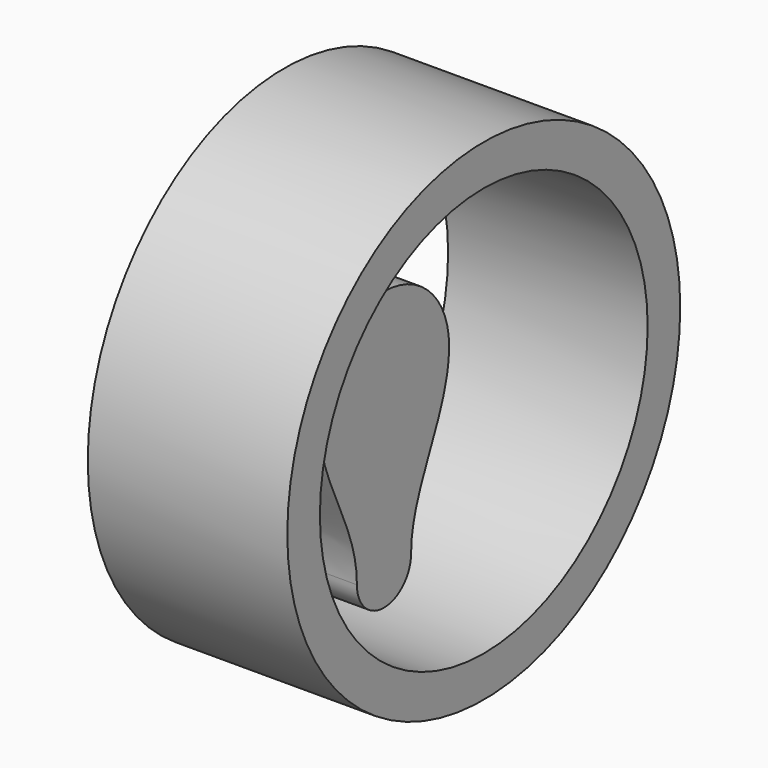
from build123d import *

# Parameters (mm, degrees)
F0_R     = 22.8209931427
F1_DEPTH = 34.544
F3_DEPTH = 51
F4_R     = 120.6073984504
F4_R_2   = 100.607397247
F5_DEPTH = 49


with BuildPart() as f1:
    # F0 (on Right) → F1 (new body)
    with BuildSketch(Plane.YZ):
        Circle(F0_R)
    extrude(amount=-F1_DEPTH)

    # F2 (on face) → F3 (join)
    with BuildSketch(Plane.YZ):
        with BuildLine():
            add(Edge.make_bspline(
                [(16.6304931045, -80.0537467003), (16.5519428961, -52.1548158816), (40.0091622509, -28.3662351914), (39.9848685014, 0)],
                knots=[0, 0, 0, 0, 83.3908221025, 83.3908221025, 83.3908221025, 83.3908221025], degree=3))
            ThreePointArc((39.9848685014, 0), (0, 39.9848685014), (-39.9848685014, 0))
            add(Edge.make_bspline(
                [(-16.6304931045, -80.0537467003), (-16.5519428961, -52.1548158816), (-40.0091622509, -28.3662351914), (-39.9848685014, 0)],
                knots=[0, 0, 0, 0, 83.3908221025, 83.3908221025, 83.3908221025, 83.3908221025], degree=3))
            ThreePointArc((-16.6304931045, -80.0537467003), (0, -96.7311293327), (16.6304931045, -80.0537467003))
        make_face()
    extrude(amount=-F3_DEPTH)


with BuildPart() as f5:
    # F4 (on face) → F5 (new body, symmetric)
    with BuildSketch(Plane.YZ):
        Circle(F4_R)
        Circle(F4_R_2, mode=Mode.SUBTRACT)
    extrude(amount=F5_DEPTH, both=True)


solid = Compound([f1.part, f5.part])
